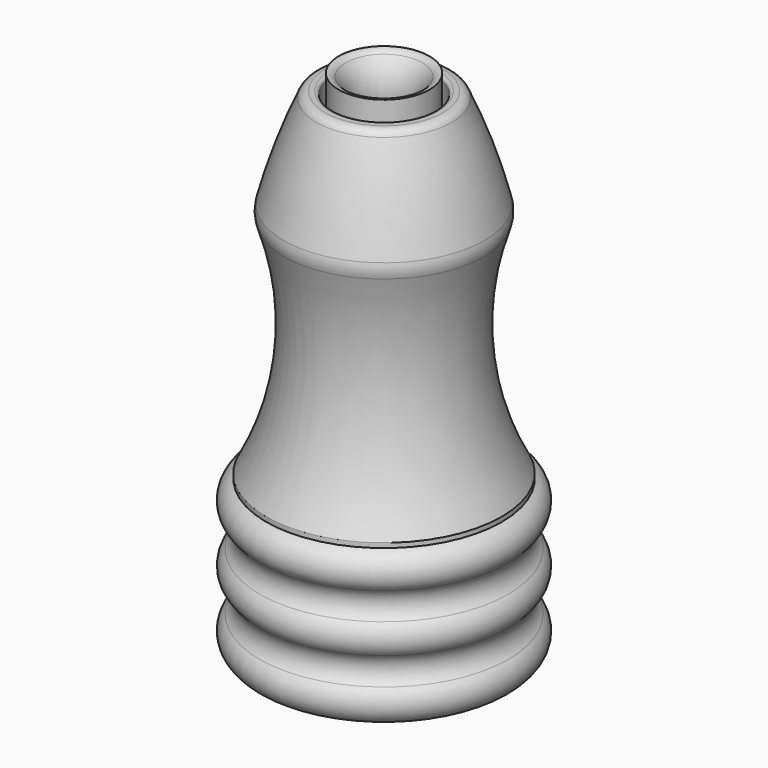
from build123d import *


# Not quite as in the source:
# - a feature names something its author has since deleted; it is built from what else it names


with BuildPart() as f1:
    # F0 (on Front) → F1 (revolve)
    with BuildSketch(Plane.XZ):
        with BuildLine():
            Line((25, 8), (25, 0))
            Line((25, 0), (36.9540249121, 0))
            Line((36.9540249121, 0), (36.9540249121, 12))
            Line((36.9540249121, 12), (36.9540249121, 18))
            Line((36.9540249121, 18), (36.9540249121, 30))
            Line((36.9540249121, 30), (36.9540249121, 36))
            Line((36.9540249121, 36), (36.9540249121, 48))
            Line((36.9540249121, 48), (36.9540249121, 49.4592389781))
            ThreePointArc((36.9540249121, 49.4592389781), (26.8120113714, 83.816301877), (31.2710027972, 119.3604378936))
            ThreePointArc((31.2710027972, 119.3604378936), (31.6978375798, 121.63115889), (31.4579349962, 123.9291598748))
            ThreePointArc((31.4579349962, 123.9291598748), (26.978512217, 138.8038130666), (21.2214044341, 153.2321271049))
            ThreePointArc((21.2214044341, 153.2321271049), (20.1145427359, 154.5195616002), (18.486105036, 155))
            Line((18.486105036, 155), (17, 155))
            ThreePointArc((17, 155), (16.2928932188, 154.7071067812), (16, 154))
            Line((16, 154), (16, 145))
            Line((16, 145), (14.25, 145))
            Line((14.25, 145), (14.25, 159.9997157952))
            ThreePointArc((14.25, 159.9997157952), (13.0109310604, 159.7130558752), (12.0019668196, 158.9388098499))
            ThreePointArc((12.0019668196, 158.9388098499), (9.2495897902, 145.9570049241), (18.5691533066, 136.5098585662))
            ThreePointArc((18.5691533066, 136.5098585662), (22.7275417245, 133.9952766931), (25.2095663012, 129.8173740816))
            ThreePointArc((25.2095663012, 129.8173740816), (26.5056514655, 125.2585186607), (27.6769844482, 120.6660271206))
            ThreePointArc((27.6769844482, 120.6660271206), (27.9522435752, 118.1190465704), (27.5713567581, 115.5857083098))
            ThreePointArc((27.5713567581, 115.5857083098), (24.3616600457, 84.3776185226), (32.0591541436, 53.963878112))
            ThreePointArc((32.0591541436, 53.963878112), (32.3885463442, 52.9608639862), (32.5, 51.9110475065))
            Line((32.5, 51.9110475065), (32.5, 8))
            Line((32.5, 8), (25, 8))
        make_face()
        with BuildLine():
            Line((36.9540249121, 12), (36.9540249121, 0))
            ThreePointArc((36.9540249121, 0), (40.8417897216, 4.7973110382), (38.9648563211, 10.68))
            ThreePointArc((38.9648563211, 10.68), (38.0210319574, 11.4338256081), (36.9540249121, 12))
        make_face()
        with BuildLine():
            Line((36.9540249121, 18), (36.9540249121, 12))
            ThreePointArc((36.9540249121, 12), (38.0210319574, 11.4338256081), (38.9648563211, 10.68))
            ThreePointArc((38.9648563211, 10.68), (37.1287006986, 15), (38.9648563211, 19.32))
            ThreePointArc((38.9648563211, 19.32), (38.0210319574, 18.5661743919), (36.9540249121, 18))
        make_face()
        with BuildLine():
            Line((36.9540249121, 30), (36.9540249121, 18))
            ThreePointArc((36.9540249121, 18), (38.0210319574, 18.5661743919), (38.9648563211, 19.32))
            ThreePointArc((38.9648563211, 19.32), (40.9540249121, 24), (38.9648563211, 28.68))
            ThreePointArc((38.9648563211, 28.68), (38.0210319574, 29.4338256081), (36.9540249121, 30))
        make_face()
        with BuildLine():
            Line((36.9540249121, 36), (36.9540249121, 30))
            ThreePointArc((36.9540249121, 30), (38.0210319574, 29.4338256081), (38.9648563211, 28.68))
            ThreePointArc((38.9648563211, 28.68), (37.1287006986, 33), (38.9648563211, 37.32))
            ThreePointArc((38.9648563211, 37.32), (38.0210319574, 36.5661743919), (36.9540249121, 36))
        make_face()
        with BuildLine():
            Line((36.9540249121, 48), (36.9540249121, 36))
            ThreePointArc((36.9540249121, 36), (38.0210319574, 36.5661743919), (38.9648563211, 37.32))
            ThreePointArc((38.9648563211, 37.32), (40.8417897216, 43.2026889618), (36.9540249121, 48))
        make_face()
    revolve(axis=Axis((0, 0, 90.2518928051), (0, 0, 1)))


solid = f1.part
